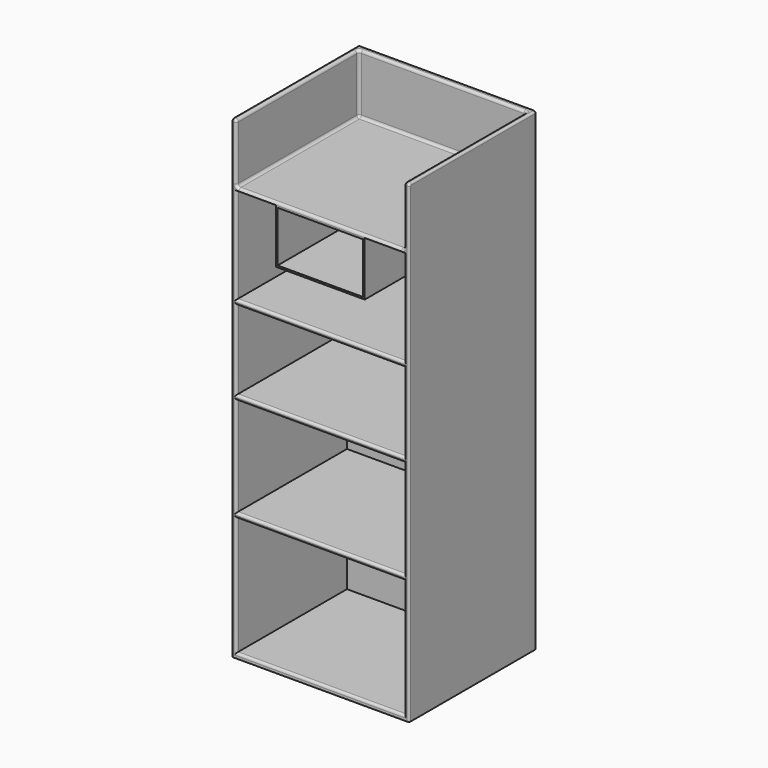
from build123d import *

# Parameters (mm, degrees)
F0_W      = 457.2
F0_H      = 406.4
F1_DEPTH  = 1219.2
F2_W      = 431.8
F2_H      = 402.8296259509
F3_DEPTH  = 152.4
F4_R      = 6.7564
F5_W      = 431.8
F5_H      = 304.8
F6_DEPTH  = 355.6
F7_W      = 431.8
F7_H      = 254
F7_H_2    = 203.2
F8_DEPTH  = 355.6
F9_R      = 6.1321024484
F10_W     = 219.456
F10_H     = 130.556
F11_DEPTH = 203.2
F12_R     = 5.08


with BuildPart() as f1:
    # F0 (on Top) → F1 (new body)
    with BuildSketch(Plane.XY):
        with Locations((-6.7284821169, -163.7329156511)):
            Rectangle(F0_W, F0_H)
    extrude(amount=-F1_DEPTH)

    # F2 (on face) → F3 (cut)
    with BuildSketch(Plane.XY):
        with Locations((-6.7284821169, -174.6477286265)):
            Rectangle(F2_W, F2_H)
    extrude(amount=-F3_DEPTH, mode=Mode.SUBTRACT)

    # F4
    f4_edges = [f1.edges().sort_by_distance(p)[0] for p in [
        (209.171518, -170.082916, -152.4),
        (-6.728482, 26.767084, -152.4),
        (209.171518, 26.767084, -76.2),
        (209.171518, -366.932916, -76.2),
        (209.171518, -170.082916, 0),
        (215.521518, -366.932916, 0),
        (-222.628482, -170.082916, -152.4),
        (-222.628482, 26.767084, -76.2),
        (-6.728482, -366.932916, -152.4),
        (-222.628482, -366.932916, -76.2),
        (-222.628482, -170.082916, 0),
        (-228.978482, -366.932916, 0),
        (-6.728482, 26.767084, 0),
    ]]
    fillet(f4_edges, radius=F4_R)

    # F5 (on face) → F6 (cut)
    with BuildSketch(Plane.XZ.offset(366.9329156511)):
        with Locations((-6.7284821169, -1054.1)):
            Rectangle(F5_W, F5_H)
    extrude(amount=-F6_DEPTH, mode=Mode.SUBTRACT)

    # F7 (on face) → F8 (cut)
    with BuildSketch(Plane.XZ.offset(366.9329156511)):
        with Locations((-6.7284821169, -762)):
            Rectangle(F7_W, F7_H)
        with Locations((-6.7284821169, -520.7)):
            Rectangle(F7_W, F7_H_2)
        Polygon((-121.0284821169, -298.8564), (-121.0284821169, -159.1564), (-222.6284821169, -159.1564), (-222.6284821169, -406.4), (209.1715178831, -406.4), (209.1715178831, -159.1564), (107.5715178831, -159.1564), (107.5715178831, -298.8564), align=None)
    extrude(amount=-F8_DEPTH, mode=Mode.SUBTRACT)

    # F9
    f9_edges = [f1.edges().sort_by_distance(p)[0] for p in [
        (-222.628482, -366.932916, -520.7),
        (209.171518, -366.932916, -520.7),
        (-222.628482, -366.932916, -282.7782),
        (209.171518, -366.932916, -282.7782),
        (209.171518, -366.932916, -762),
        (-222.628482, -366.932916, -762),
        (-222.628482, -366.932916, -1054.1),
        (209.171518, -366.932916, -1054.1),
        (-6.728482, -366.932916, -1206.5),
        (-6.728482, -366.932916, -889),
        (-6.728482, -366.932916, -901.7),
        (-6.728482, -366.932916, -635),
        (-6.728482, -366.932916, -622.3),
        (-6.728482, -366.932916, -419.1),
        (-6.728482, -366.932916, -406.4),
    ]]
    fillet(f9_edges, radius=F9_R)

    # F10 (on face) → F11 (cut)
    with BuildSketch(Plane.XZ.offset(366.9329156511)):
        with Locations((-6.7284821169, -229.0064)):
            Rectangle(F10_W, F10_H)
    extrude(amount=-F11_DEPTH, mode=Mode.SUBTRACT)

    # F12
    f12_edges = [f1.edges().sort_by_distance(p)[0] for p in [
        (-235.328482, -366.932916, -612.9782),
        (221.871518, -366.932916, -612.9782),
        (221.871518, -160.354716, 0),
        (-235.328482, -160.354716, 0),
        (221.871518, -364.954012, -1.978904),
        (-235.328482, -364.954012, -1.978904),
    ]]
    fillet(f12_edges, radius=F12_R)


solid = f1.part
